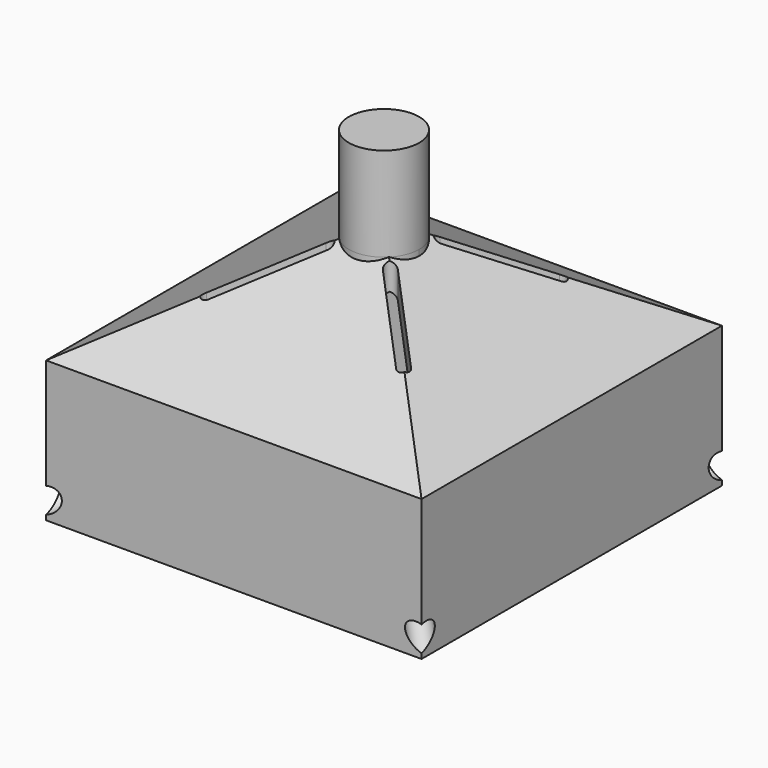
from build123d import *

# Parameters (mm, degrees)
F0_W           = 203.2
F0_H           = 203.2
F1_DEPTH       = 127
F2_W           = 152.4
F2_H           = 152.4
F3_DEPTH       = 76.2
F4_W           = 152.4
F4_H           = 152.4
F6_C1_SIZE2    = 87.9881810245
F6_C1_SIZE     = 50.8
F6_C2_SIZE2    = 87.9881810245
F6_C2_SIZE     = 50.8
F6_C3_SIZE2    = 50.8
F6_C3_SIZE     = 87.9881810245
F6_C4_SIZE2    = 87.9881810245
F6_C4_SIZE     = 50.8
F8_DEPTH       = 127
F10_R          = 6.35
F11_DEPTH      = 76.2
F15_R          = 6.35
F16_DEPTH      = 127
F17_R          = 6.35
F18_DEPTH      = 127
F19_R          = 6.35
F20_DEPTH      = 127
F21_R          = 19.05
F22_DEPTH      = 50.8
F22_DEPTH_BACK = 12.7


# Not quite as in the source:
# - an extrude whose draft closes it to a point is written as a loft to that point


with BuildPart() as f1:
    # F0 (on Top) → F1 (new body)
    with BuildSketch(Plane.XY):
        Rectangle(F0_W, F0_H)
    extrude(amount=F1_DEPTH)

    # F2 (on face) → F3 (cut)
    with BuildSketch(Plane.XY):
        Rectangle(F2_W, F2_H)
    extrude(amount=F3_DEPTH, mode=Mode.SUBTRACT)

    # F4 (on face) → F5 section 0
    with BuildSketch(Plane(origin=(0, 0, 76.2), x_dir=(1, 0, 0), z_dir=(0, 0, -1)), mode=Mode.PRIVATE) as f5_s0:
        Rectangle(F4_W, F4_H)
    loft([f5_s0.sketch, Vertex(0, 0, 120.1940905122)], ruled=True, mode=Mode.SUBTRACT)

    # F6: chamfer of 50.8 x 87.9881810245 on 4 edges, made by hand

    # F6_c1
    f6_c1_edges = [f1.edges().sort_by_distance(p)[0] for p in [
        (0, -101.6, 127),
    ]]
    f6_c1_side = f1.faces().sort_by_distance((0, -101.6, 125.984))[0]
    chamfer(f6_c1_edges, length=F6_C1_SIZE, length2=F6_C1_SIZE2, reference=f6_c1_side)

    # F6_c2
    f6_c2_edges = [f1.edges().sort_by_distance(p)[0] for p in [
        (-101.6, 43.9940905122, 127),
    ]]
    f6_c2_side = f1.faces().sort_by_distance((-101.6, 43.9940905122, 125.984))[0]
    chamfer(f6_c2_edges, length=F6_C2_SIZE, length2=F6_C2_SIZE2, reference=f6_c2_side)

    # F6_c3
    f6_c3_edges = [f1.edges().sort_by_distance(p)[0] for p in [
        (101.6, 43.9940905122, 127),
    ]]
    f6_c3_side = f1.faces().sort_by_distance((100.584, 43.9940905122, 127))[0]
    chamfer(f6_c3_edges, length=F6_C3_SIZE, length2=F6_C3_SIZE2, reference=f6_c3_side)

    # F6_c4
    f6_c4_edges = [f1.edges().sort_by_distance(p)[0] for p in [
        (0, 101.6, 127),
    ]]
    f6_c4_side = f1.faces().sort_by_distance((0, 101.6, 125.984))[0]
    chamfer(f6_c4_edges, length=F6_C4_SIZE, length2=F6_C4_SIZE2, reference=f6_c4_side)

    # F7 (on Top) → F8 (cut, through all)
    with BuildSketch(Plane.XY):
        with BuildLine():
            Line((-19.3939794208, -14.9038513603), (-55.3150039051, -50.8248758446))
            ThreePointArc((-55.3150039051, -50.8248758446), (-55.3150039051, -55.3150039051), (-50.8248758446, -55.3150039051))
            Line((-50.8248758446, -55.3150039051), (-14.9038513603, -19.3939794208))
            ThreePointArc((-14.9038513603, -19.3939794208), (-14.9038513603, -14.9038513603), (-19.3939794208, -14.9038513603))
        make_face()
        with BuildLine():
            Line((-55.3150039051, 50.8248758446), (-19.3939794208, 14.9038513603))
            ThreePointArc((-19.3939794208, 14.9038513603), (-14.9038513603, 14.9038513603), (-14.9038513603, 19.3939794208))
            Line((-14.9038513603, 19.3939794208), (-50.8248758446, 55.3150039051))
            ThreePointArc((-50.8248758446, 55.3150039051), (-55.3150039051, 55.3150039051), (-55.3150039051, 50.8248758446))
        make_face()
        with BuildLine():
            Line((50.8248758446, 55.3150039051), (14.9038513603, 19.3939794208))
            ThreePointArc((14.9038513603, 19.3939794208), (14.9038513603, 14.9038513603), (19.3939794208, 14.9038513603))
            Line((19.3939794208, 14.9038513603), (55.3150039051, 50.8248758446))
            ThreePointArc((55.3150039051, 50.8248758446), (55.3150039051, 55.3150039051), (50.8248758446, 55.3150039051))
        make_face()
        with BuildLine():
            Line((55.3150039051, -50.8248758446), (19.3939794208, -14.9038513603))
            ThreePointArc((19.3939794208, -14.9038513603), (14.9038513603, -14.9038513603), (14.9038513603, -19.3939794208))
            Line((14.9038513603, -19.3939794208), (50.8248758446, -55.3150039051))
            ThreePointArc((50.8248758446, -55.3150039051), (55.3150039051, -55.3150039051), (55.3150039051, -50.8248758446))
        make_face()
    extrude(amount=F8_DEPTH, mode=Mode.SUBTRACT)

    # F10 (on face) → F11 (cut)
    with BuildSketch(Plane(origin=(87.0857142857, -87.0857142857, -50.2789605854), x_dir=(0.755928946, 0.5669467095, 0.3273268354), z_dir=(0.6546536707, -0.6546536707, -0.377964473))):
        with Locations((22.3436848712, 59.1158335421)):
            Circle(F10_R)
    extrude(amount=-F11_DEPTH, mode=Mode.SUBTRACT)

    # F15 (on face) → F16 (cut)
    with BuildSketch(Plane(origin=(-87.0857142857, -87.0857142857, -50.2789605854), x_dir=(0.5669467095, -0.755928946, 0.3273268354), z_dir=(-0.6546536707, -0.6546536707, -0.377964473))):
        with Locations((22.0481136328, 59.221623296)):
            Circle(F15_R)
    extrude(amount=-F16_DEPTH, mode=Mode.SUBTRACT)

    # F17 (on face) → F18 (cut)
    with BuildSketch(Plane(origin=(-87.0857142857, 87.0857142857, -50.2789605854), x_dir=(-0.755928946, -0.5669467095, 0.3273268354), z_dir=(-0.6546536707, 0.6546536707, -0.377964473))):
        with Locations((22.3436848712, 59.1158335421)):
            Circle(F17_R)
    extrude(amount=-F18_DEPTH, mode=Mode.SUBTRACT)

    # F19 (on face) → F20 (cut)
    with BuildSketch(Plane(origin=(87.0857142857, 87.0857142857, -50.2789605854), x_dir=(-0.755928946, 0.5669467095, -0.3273268354), z_dir=(0.6546536707, 0.6546536707, -0.377964473))):
        with Locations((-22.3436848712, 59.1158335421)):
            Circle(F19_R)
    extrude(amount=-F20_DEPTH, mode=Mode.SUBTRACT)

    # F21 (on face) → F22 (join, two sides)
    with BuildSketch(Plane.XY.offset(127)) as f22_sk:
        Circle(F21_R)
    extrude(amount=F22_DEPTH)
    extrude(f22_sk.sketch, amount=-F22_DEPTH_BACK)


solid = f1.part
